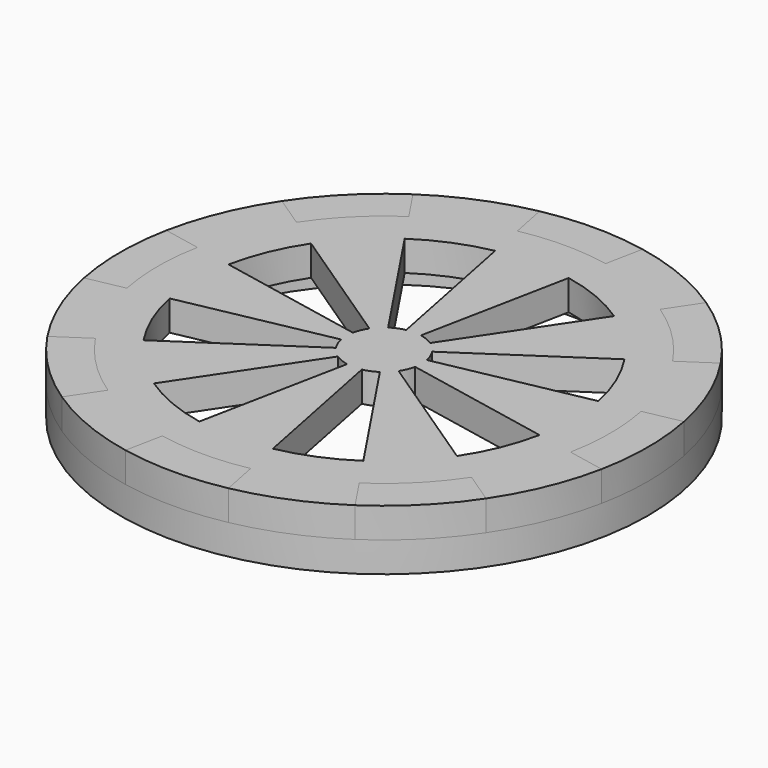
from build123d import *

# Parameters (mm, degrees)
F0_R     = 35
F0_R_2   = 30
F1_DEPTH = 4
F3_DEPTH = 4
F5_DEPTH = 4


# Not quite as in the source:
# - after a boolean that leaves OpenCascade's solid faulty, fix() repairs it


with BuildPart() as f1:
    # F0 (on Top) → F1 (new body)
    with BuildSketch(Plane.XY):
        Circle(F0_R)
        Circle(F0_R_2, mode=Mode.SUBTRACT)
    extrude(amount=F1_DEPTH)

    # F2 (on face) → F3 (join)
    with BuildSketch(Plane.XY.offset(4)):
        with BuildLine():
            Line((-6.8281612706, 34.3274848141), (-5.8527096605, 29.4235584121))
            ThreePointArc((-5.8527096605, 29.4235584121), (0, 30), (5.8527096605, 29.4235584121))
            Line((5.8527096605, 29.4235584121), (6.8281612706, 34.3274848141))
            ThreePointArc((6.8281612706, 34.3274848141), (0, 35), (-6.8281612706, 34.3274848141))
        make_face()
        with BuildLine():
            ThreePointArc((-24.9440883691, 16.6671069906), (-21.2132034356, 21.2132034356), (-16.6671069906, 24.9440883691))
            Line((-16.6671069906, 24.9440883691), (-19.4449581557, 29.1014364306))
            ThreePointArc((-19.4449581557, 29.1014364306), (-24.7487373415, 24.7487373415), (-29.1014364306, 19.4449581557))
            Line((-29.1014364306, 19.4449581557), (-24.9440883691, 16.6671069906))
        make_face()
        with BuildLine():
            ThreePointArc((-29.4235584121, -5.8527096605), (-30, 0), (-29.4235584121, 5.8527096605))
            Line((-29.4235584121, 5.8527096605), (-34.3274848141, 6.8281612706))
            ThreePointArc((-34.3274848141, 6.8281612706), (-35, 0), (-34.3274848141, -6.8281612706))
            Line((-34.3274848141, -6.8281612706), (-29.4235584121, -5.8527096605))
        make_face()
        with BuildLine():
            ThreePointArc((-16.6671069906, -24.9440883691), (-21.2132034356, -21.2132034356), (-24.9440883691, -16.6671069906))
            Line((-24.9440883691, -16.6671069906), (-29.1014364306, -19.4449581557))
            ThreePointArc((-29.1014364306, -19.4449581557), (-24.7487373415, -24.7487373415), (-19.4449581557, -29.1014364306))
            Line((-19.4449581557, -29.1014364306), (-16.6671069906, -24.9440883691))
        make_face()
        with BuildLine():
            ThreePointArc((5.8527096605, -29.4235584121), (0, -30), (-5.8527096605, -29.4235584121))
            Line((-5.8527096605, -29.4235584121), (-6.8281612706, -34.3274848141))
            ThreePointArc((-6.8281612706, -34.3274848141), (0, -35), (6.8281612706, -34.3274848141))
            Line((6.8281612706, -34.3274848141), (5.8527096605, -29.4235584121))
        make_face()
        with BuildLine():
            ThreePointArc((24.9440883691, -16.6671069906), (21.2132034356, -21.2132034356), (16.6671069906, -24.9440883691))
            Line((16.6671069906, -24.9440883691), (19.4449581557, -29.1014364306))
            ThreePointArc((19.4449581557, -29.1014364306), (24.7487373415, -24.7487373415), (29.1014364306, -19.4449581557))
            Line((29.1014364306, -19.4449581557), (24.9440883691, -16.6671069906))
        make_face()
        with BuildLine():
            ThreePointArc((29.4235584121, 5.8527096605), (30, 0), (29.4235584121, -5.8527096605))
            Line((29.4235584121, -5.8527096605), (34.3274848141, -6.8281612706))
            ThreePointArc((34.3274848141, -6.8281612706), (35, 0), (34.3274848141, 6.8281612706))
            Line((34.3274848141, 6.8281612706), (29.4235584121, 5.8527096605))
        make_face()
        with BuildLine():
            ThreePointArc((16.6671069906, 24.9440883691), (21.2132034356, 21.2132034356), (24.9440883691, 16.6671069906))
            Line((24.9440883691, 16.6671069906), (29.1014364306, 19.4449581557))
            ThreePointArc((29.1014364306, 19.4449581557), (24.7487373415, 24.7487373415), (19.4449581557, 29.1014364306))
            Line((19.4449581557, 29.1014364306), (16.6671069906, 24.9440883691))
        make_face()
    extrude(amount=F3_DEPTH)

    add(f1.part.fix(), mode=Mode.REPLACE)


with BuildPart() as f5:
    # F4 (on face) → F5 (new body)
    with BuildSketch(Plane.XY.offset(4)):
        with BuildLine():
            Line((-24.9440883691, 16.6671069906), (-29.1014364306, 19.4449581557))
            ThreePointArc((-29.1014364306, 19.4449581557), (-32.3357836379, 13.3939201328), (-34.3274848141, 6.8281612706))
            Line((-34.3274848141, 6.8281612706), (-29.4235584121, 5.8527096605))
            ThreePointArc((-29.4235584121, 5.8527096605), (-30, 0), (-29.4235584121, -5.8527096605))
            Line((-29.4235584121, -5.8527096605), (-34.3274848141, -6.8281612706))
            ThreePointArc((-34.3274848141, -6.8281612706), (-32.3357836379, -13.3939201328), (-29.1014364306, -19.4449581557))
            Line((-29.1014364306, -19.4449581557), (-24.9440883691, -16.6671069906))
            ThreePointArc((-24.9440883691, -16.6671069906), (-21.2132034356, -21.2132034356), (-16.6671069906, -24.9440883691))
            Line((-16.6671069906, -24.9440883691), (-19.4449581557, -29.1014364306))
            ThreePointArc((-19.4449581557, -29.1014364306), (-13.3939201328, -32.3357836379), (-6.8281612706, -34.3274848141))
            Line((-6.8281612706, -34.3274848141), (-5.8527096605, -29.4235584121))
            ThreePointArc((-5.8527096605, -29.4235584121), (0, -30), (5.8527096605, -29.4235584121))
            Line((5.8527096605, -29.4235584121), (6.8281612706, -34.3274848141))
            ThreePointArc((6.8281612706, -34.3274848141), (13.3939201328, -32.3357836379), (19.4449581557, -29.1014364306))
            Line((19.4449581557, -29.1014364306), (16.6671069906, -24.9440883691))
            ThreePointArc((16.6671069906, -24.9440883691), (21.2132034356, -21.2132034356), (24.9440883691, -16.6671069906))
            Line((24.9440883691, -16.6671069906), (29.1014364306, -19.4449581557))
            ThreePointArc((29.1014364306, -19.4449581557), (32.3357836379, -13.3939201328), (34.3274848141, -6.8281612706))
            Line((34.3274848141, -6.8281612706), (29.4235584121, -5.8527096605))
            ThreePointArc((29.4235584121, -5.8527096605), (30, 0), (29.4235584121, 5.8527096605))
            Line((29.4235584121, 5.8527096605), (34.3274848141, 6.8281612706))
            ThreePointArc((34.3274848141, 6.8281612706), (32.3357836379, 13.3939201328), (29.1014364306, 19.4449581557))
            Line((29.1014364306, 19.4449581557), (24.9440883691, 16.6671069906))
            ThreePointArc((24.9440883691, 16.6671069906), (21.2132034356, 21.2132034356), (16.6671069906, 24.9440883691))
            Line((16.6671069906, 24.9440883691), (19.4449581557, 29.1014364306))
            ThreePointArc((19.4449581557, 29.1014364306), (13.3939201328, 32.3357836379), (6.8281612706, 34.3274848141))
            Line((6.8281612706, 34.3274848141), (5.8527096605, 29.4235584121))
            ThreePointArc((5.8527096605, 29.4235584121), (0, 30), (-5.8527096605, 29.4235584121))
            Line((-5.8527096605, 29.4235584121), (-6.8281612706, 34.3274848141))
            ThreePointArc((-6.8281612706, 34.3274848141), (-13.3939201328, 32.3357836379), (-19.4449581557, 29.1014364306))
            Line((-19.4449581557, 29.1014364306), (-16.6671069906, 24.9440883691))
            ThreePointArc((-16.6671069906, 24.9440883691), (-21.2132034356, 21.2132034356), (-24.9440883691, 16.6671069906))
        make_face()
        with BuildLine():
            ThreePointArc((-2.7778511776, -4.1573480531), (-1.913417175, -4.6193976571), (-0.9754516234, -4.9039263994))
            Line((-0.9754516234, -4.9039263994), (-4.8772581169, -24.5196319969))
            ThreePointArc((-4.8772581169, -24.5196319969), (-9.5670858752, -23.0969882854), (-13.8892558881, -20.7867402657))
            Line((-13.8892558881, -20.7867402657), (-2.7778511776, -4.1573480531))
        make_face(mode=Mode.SUBTRACT)
        with BuildLine():
            ThreePointArc((-4.9039264055, -0.9754515924), (-4.6193976692, -1.9134171458), (-4.1573480707, -2.7778511513))
            Line((-4.1573480707, -2.7778511513), (-20.7867403536, -13.8892557566))
            ThreePointArc((-20.7867403536, -13.8892557566), (-23.0969883459, -9.5670857291), (-24.5196320277, -4.8772579618))
            Line((-24.5196320277, -4.8772579618), (-4.9039264055, -0.9754515924))
        make_face(mode=Mode.SUBTRACT)
        with BuildLine():
            ThreePointArc((0.9754515983, -4.9039264044), (1.9134171514, -4.6193976669), (2.7778511563, -4.1573480674))
            Line((2.7778511563, -4.1573480674), (13.8892557817, -20.7867403369))
            ThreePointArc((13.8892557817, -20.7867403369), (9.5670857569, -23.0969883344), (4.8772579913, -24.5196320218))
            Line((4.8772579913, -24.5196320218), (0.9754515983, -4.9039264044))
        make_face(mode=Mode.SUBTRACT)
        with BuildLine():
            Line((20.7867402825, -13.8892558631), (4.1573480565, -2.7778511726))
            ThreePointArc((4.1573480565, -2.7778511726), (4.6193976594, -1.9134171695), (4.9039264005, -0.9754516175))
            Line((4.9039264005, -0.9754516175), (24.5196320027, -4.8772580873))
            ThreePointArc((24.5196320027, -4.8772580873), (23.0969882969, -9.5670858474), (20.7867402825, -13.8892558631))
        make_face(mode=Mode.SUBTRACT)
        with BuildLine():
            ThreePointArc((-4.1573480498, 2.7778511826), (-4.6193976548, 1.9134171806), (-4.9039263982, 0.9754516293))
            Line((-4.9039263982, 0.9754516293), (-24.519631991, 4.8772581464))
            ThreePointArc((-24.519631991, 4.8772581464), (-23.0969882739, 9.5670859031), (-20.786740249, 13.8892559132))
            Line((-20.786740249, 13.8892559132), (-4.1573480498, 2.7778511826))
        make_face(mode=Mode.SUBTRACT)
        with BuildLine():
            ThreePointArc((-13.8892557316, 20.7867403703), (-9.5670857569, 23.0969883344), (-4.8772580504, 24.5196320101))
            Line((-4.8772580504, 24.5196320101), (-0.9754516101, 4.903926402))
            ThreePointArc((-0.9754516101, 4.903926402), (-1.9134171514, 4.6193976669), (-2.7778511463, 4.1573480741))
            Line((-2.7778511463, 4.1573480741), (-13.8892557316, 20.7867403703))
        make_face(mode=Mode.SUBTRACT)
        with BuildLine():
            ThreePointArc((4.9039264032, 0.9754516042), (4.6193976646, 1.913417157), (4.157348064, 2.7778511613))
            Line((4.157348064, 2.7778511613), (20.7867403201, 13.8892558067))
            ThreePointArc((20.7867403201, 13.8892558067), (23.0969883229, 9.5670857848), (24.519632016, 4.8772580209))
            Line((24.519632016, 4.8772580209), (4.9039264032, 0.9754516042))
        make_face(mode=Mode.SUBTRACT)
        with BuildLine():
            ThreePointArc((2.7778511676, 4.1573480598), (1.9134171639, 4.6193976617), (0.9754516116, 4.9039264017))
            Line((0.9754516116, 4.9039264017), (4.8772580578, 24.5196320086))
            ThreePointArc((4.8772580578, 24.5196320086), (9.5670858196, 23.0969883085), (13.889255838, 20.7867402992))
            Line((13.889255838, 20.7867402992), (2.7778511676, 4.1573480598))
        make_face(mode=Mode.SUBTRACT)
    extrude(amount=F5_DEPTH)


solid = Compound([f1.part, f5.part])
